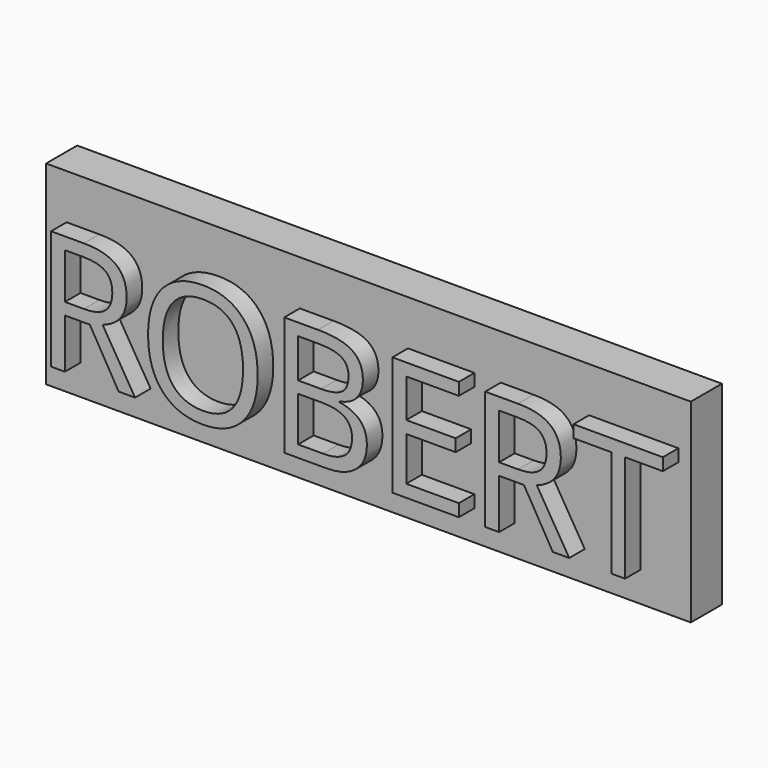
from build123d import *

# Parameters (mm, degrees)
F0_W         = 84.2210602588
F0_H         = 25.4
F1_DEPTH     = 5.08
F2_TEXT_SIZE = 21.8056607991
F3_DEPTH     = 2.54


# Not quite as in the source:
# - Text() gives the source's letters only with a copy of the font that has no kerning and outlines rounded to 1/6400 em; it was checked with that copy


with BuildPart() as f1:
    # F0 (on Front) → F1 (new body)
    with BuildSketch(Plane.XZ):
        Rectangle(F0_W, F0_H)
    extrude(amount=F1_DEPTH)

    # F2 (on face) → F3 (join)
    with BuildSketch(Plane.XZ.offset(5.08)):
        with Locations((-41.5649451315, -8.7558114901)):
            Text('ROBERT', F2_TEXT_SIZE, font='Open Sans', text_align=(TextAlign.LEFT, TextAlign.BOTTOM))
    extrude(amount=F3_DEPTH)


solid = f1.part
